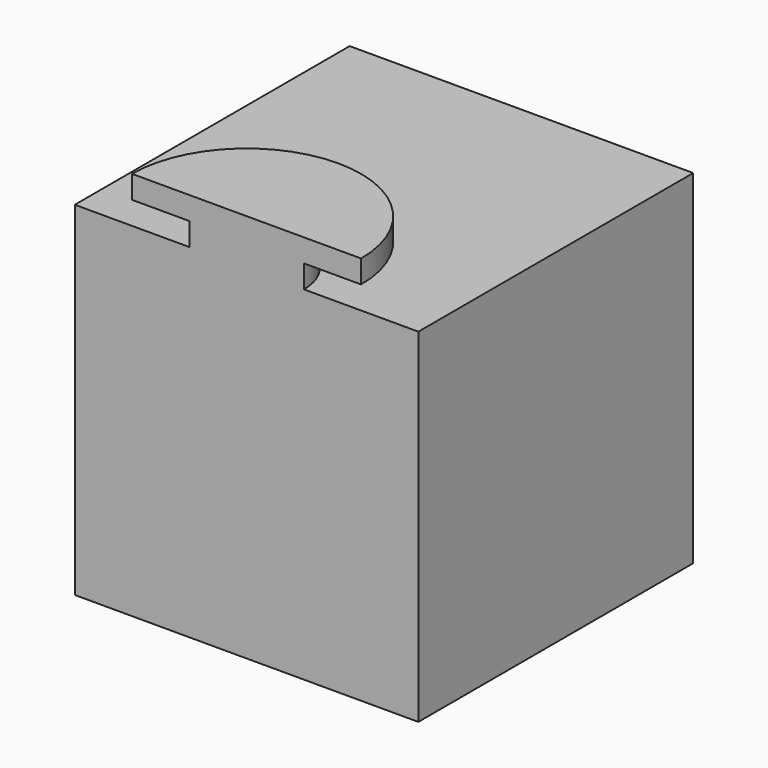
from build123d import *

# Parameters (mm, degrees)
F0_W     = 19.05
F0_H     = 19.05
F1_DEPTH = 19.05
F3_DEPTH = 1.27
F5_DEPTH = 1.27


with BuildPart() as f1:
    # F0 (on Front) → F1 (new body)
    with BuildSketch(Plane.XZ):
        with Locations((-42.3251483589, 44.0142245242)):
            Rectangle(F0_W, F0_H)
    extrude(amount=F1_DEPTH)

    # F2 (on face) → F3 (join)
    with BuildSketch(Plane.XY.offset(53.5392245242)):
        with BuildLine():
            Line((-45.5001483589, -19.05), (-39.1501483589, -19.05))
            ThreePointArc((-39.1501483589, -19.05), (-42.3251483589, -15.875), (-45.5001483589, -19.05))
        make_face()
    extrude(amount=F3_DEPTH)

    # F4 (on face) → F5 (join)
    with BuildSketch(Plane.XY.offset(54.8092245242)):
        with BuildLine():
            Line((-45.5001483589, -19.05), (-39.1501483589, -19.05))
            ThreePointArc((-39.1501483589, -19.05), (-42.3251483589, -15.875), (-45.5001483589, -19.05))
        make_face()
        with BuildLine():
            Line((-39.1501483589, -19.05), (-35.9751483589, -19.05))
            ThreePointArc((-35.9751483589, -19.05), (-42.3251483589, -12.7), (-48.6751483589, -19.05))
            Line((-48.6751483589, -19.05), (-45.5001483589, -19.05))
            ThreePointArc((-45.5001483589, -19.05), (-42.3251483589, -15.875), (-39.1501483589, -19.05))
        make_face()
    extrude(amount=F5_DEPTH)


solid = f1.part
